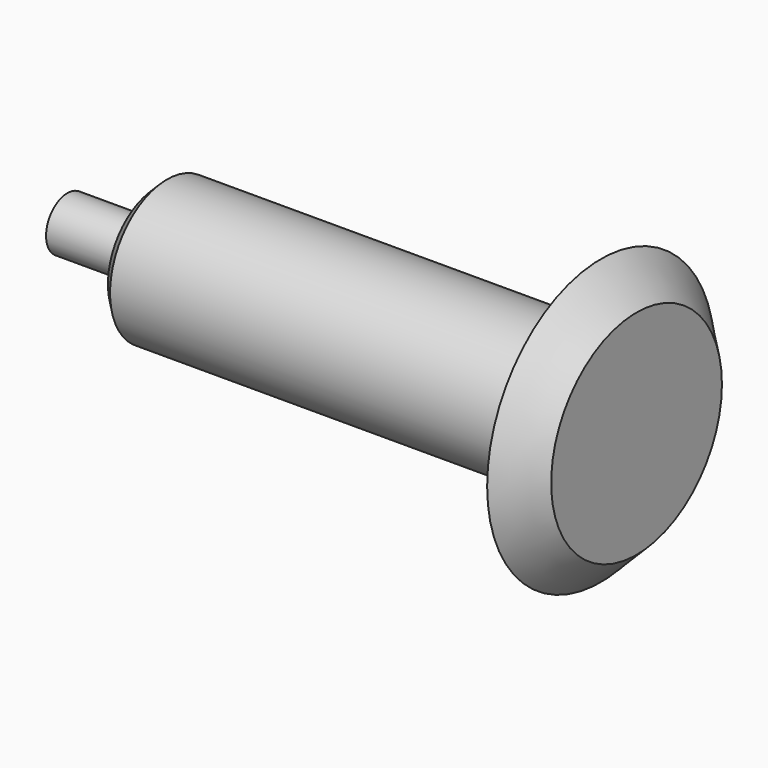
from build123d import *

# Parameters (mm, degrees)
F2_SIZE = 3
F3_SIZE = 9.99999


# Not quite as in the source:
# - a fillet or chamfer is up to 0.001 mm smaller than in the source, because OpenCascade refuses the exact size


with BuildPart() as f1:
    # F0 (on Top) → F1 (revolve)
    with BuildSketch(Plane.XY):
        Polygon((0, 7.5), (0, 0), (160, 0), (160, 40), (150, 40), (150, 20), (25, 20), (25, 7.5), align=None)
    revolve(axis=Axis((80, 0, 0), (-1, 0, 0)))

    # F2
    f2_edges = [f1.edges().sort_by_distance(p)[0] for p in [
        (25, -20, 0),
    ]]
    chamfer(f2_edges, length=F2_SIZE)

    # F3 (size 10 in the source; OpenCascade refuses exactly that, so slightly less here)
    f3_edges = [f1.edges().sort_by_distance(p)[0] for p in [
        (150, -20, 0),
        (160, -40, 0),
    ]]
    chamfer(f3_edges, length=F3_SIZE)


solid = f1.part
